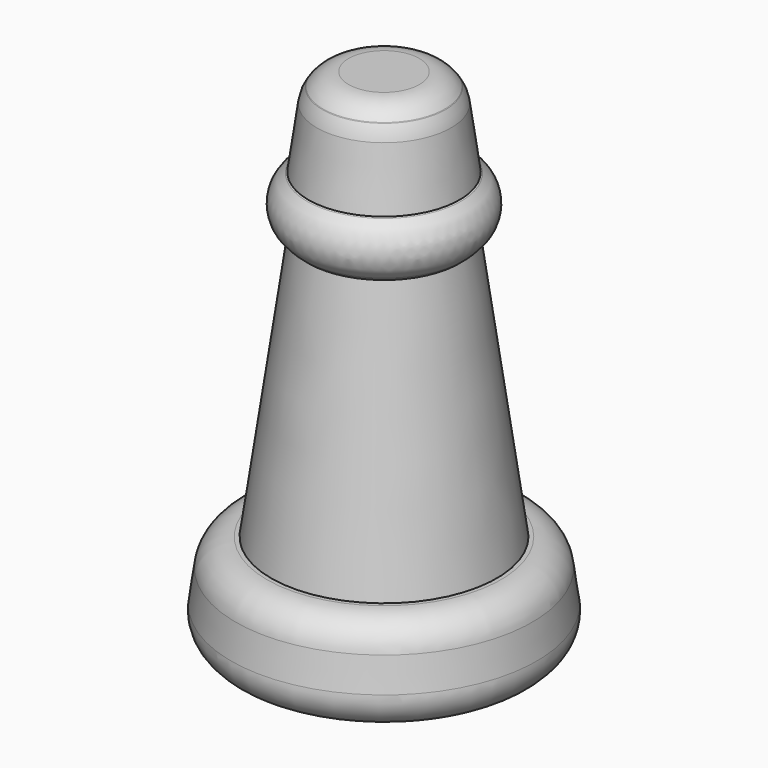
from build123d import *

# Parameters (mm, degrees)
F2_R = 1.27
F3_R = 1.27


with BuildPart() as f1:
    # F0 (on Front) → F1 (revolve)
    with BuildSketch(Plane.XZ):
        Polygon((-5.8082070693, 3.8550570151), (-6.35, 0), (0, 0), (0, 20.32), (-2.071337691, 20.32), (-2.6532195265, 19.5133350633), (-3.0396357876, 16.7638404987), (-4.5382070693, 15.8119048065), (-3.0396357876, 14.5179457392), (-4.5382070693, 3.8550570151), align=None)
    revolve(axis=Axis((0, 0, 10.16), (0, 0, -1)))

    # F2
    f2_edges = [f1.edges().sort_by_distance(p)[0] for p in [
        (2.071338, 0, 20.32),
        (2.65322, 0, 19.513335),
        (-2.362279, 0, 19.916668),
    ]]
    fillet(f2_edges, radius=F2_R)

    # F3
    f3_edges = [f1.edges().sort_by_distance(p)[0] for p in [
        (5.808207, 0, 3.855057),
        (1.421509, 0, 20.32),
        (4.538207, 0, 15.811905),
        (6.35, 0, 0),
    ]]
    fillet(f3_edges, radius=F3_R)


solid = f1.part
